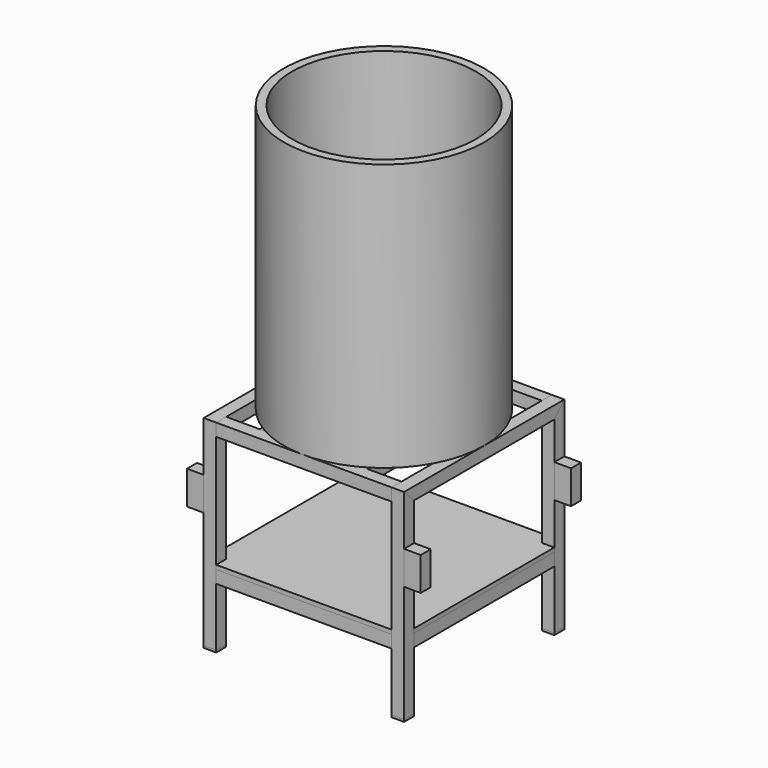
from build123d import *

# Parameters (mm, degrees)
F0_R           = 304.8
F1_DEPTH       = 812.8
F2_W           = 38.1
F2_H           = 38.1
F2_W_2         = 30.48
F2_H_2         = 30.48
F3_DEPTH       = 304.8
F5_DEPTH       = 38.1
F8_W           = 38.1
F8_H           = 38.1
F8_W_2         = 30.48
F8_H_2         = 30.48
F9_REACH       = 1476.2825367264
F12_W          = 38.1
F12_H          = 38.1
F12_W_2        = 30.48
F12_H_2        = 30.48
F13_DEPTH      = 266.7
F13_DEPTH_BACK = 266.7
F17_W          = 38.1
F17_H          = 38.1
F17_W_2        = 30.48
F17_H_2        = 30.48
F18_DEPTH      = 266.7
F18_DEPTH_BACK = 266.7
F20_W          = 38.1
F20_H          = 38.1
F20_W_2        = 30.48
F20_H_2        = 30.48
F21_DEPTH      = 266.7
F21_DEPTH_BACK = 266.7
F24_DEPTH      = 12.7
F25_W          = 38.1
F25_H          = 38.1
F25_R          = 6.35
F26_DEPTH      = 6.35
F29_R          = 279.4
F30_DEPTH      = 759.46
F31_W          = 38.1
F31_H          = 101.6
F32_DEPTH      = 50.8


with BuildPart() as f1:
    # F0 (on Top) → F1 (new body)
    with BuildSketch(Plane.XY):
        Circle(F0_R)
    extrude(amount=F1_DEPTH)

    # F29 (on face) → F30 (cut)
    with BuildSketch(Plane.XY.offset(812.8)):
        Circle(F29_R)
    extrude(amount=-F30_DEPTH, mode=Mode.SUBTRACT)


with BuildPart() as f3:
    # F2 (on Front) → F3 (new body, symmetric)
    with BuildSketch(Plane.XZ):
        with Locations((285.75, -19.05)):
            Rectangle(F2_W, F2_H)
        with Locations((285.75, -19.05)):
            Rectangle(F2_W_2, F2_H_2, mode=Mode.SUBTRACT)
    extrude(amount=F3_DEPTH, both=True)

    # F4 (on face) → F5 (cut, through all)
    with BuildSketch(Plane.YZ.offset(304.8)):
        Polygon((-266.7, -38.1), (-304.8, 0), (-315.9340023994, 0), (-315.9340023994, -51.912445575), (-266.7, -51.912445575), align=None)
        Polygon((315.9340023994, -51.912445575), (315.9340023994, 0), (304.8, 0), (266.7, -38.1), (266.7, -51.912445575), align=None)
    extrude(amount=-F5_DEPTH, mode=Mode.SUBTRACT)


with BuildPart() as f6_1:
    # F6: instance of F3
    add(f3.part.mirror(Plane.YZ))


with BuildPart() as f9:
    f9_end = f3.part.faces().sort_by_distance((285.75, -267.166627796, -37.633372204))[0]
    # F8 (on offset) → F9 (new body, up to a face of F3 that its end follows)
    with BuildSketch(Plane.XY.offset(-609.6)):
        with Locations((285.75, -285.75)):
            Rectangle(F8_W, F8_H)
        with Locations((285.75, -285.75)):
            Rectangle(F8_W_2, F8_H_2, mode=Mode.SUBTRACT)
    f9_long = extrude(amount=F9_REACH, mode=Mode.PRIVATE)
    add(split(f9_long, bisect_by=f9_end, keep=Keep.TOP, mode=Mode.PRIVATE))


with BuildPart() as f10_1:
    # F10: instance of F9
    add(f9.part.mirror(Plane.XZ))


with BuildPart() as f11_1:
    # F11: instance of F9
    add(f9.part.mirror(Plane.YZ))


with BuildPart() as f11_2:
    # F11: instance of F10_1
    add(f10_1.part.mirror(Plane.YZ))


with BuildPart() as f13:
    # F12 (on Right) → F13 (new body, two sides)
    with BuildSketch(Plane.YZ) as f13_sk:
        with Locations((-285.75, -19.05)):
            Rectangle(F12_W, F12_H)
        with Locations((-285.75, -19.05)):
            Rectangle(F12_W_2, F12_H_2, mode=Mode.SUBTRACT)
    extrude(amount=F13_DEPTH)
    extrude(f13_sk.sketch, amount=-F13_DEPTH_BACK)


with BuildPart() as f14_1:
    # F14: instance of F13
    add(f13.part.mirror(Plane.XZ))


with BuildPart() as f16_1:
    # F16: instance of F13
    add(f13.part.mirror(Plane(origin=(0, -285.75, -215.9), x_dir=(1, 0, 0), z_dir=(0, 0, -1))))


with BuildPart() as f16_2:
    # F16: instance of F14_1
    add(f14_1.part.mirror(Plane(origin=(0, -285.75, -215.9), x_dir=(1, 0, 0), z_dir=(0, 0, -1))))


with BuildPart() as f18:
    # F17 (on Front) → F18 (new body, two sides)
    with BuildSketch(Plane.XZ) as f18_sk:
        with Locations((285.75, -412.75)):
            Rectangle(F17_W, F17_H)
        with Locations((285.75, -412.75)):
            Rectangle(F17_W_2, F17_H_2, mode=Mode.SUBTRACT)
    extrude(amount=F18_DEPTH)
    extrude(f18_sk.sketch, amount=-F18_DEPTH_BACK)


with BuildPart() as f19_1:
    # F19: instance of F18
    add(f18.part.mirror(Plane.YZ))


with BuildPart() as f21:
    # F20 (on Front) → F21 (new body, two sides)
    with BuildSketch(Plane.XZ) as f21_sk:
        with Locations((-146.05, -19.05)):
            Rectangle(F20_W, F20_H)
        with Locations((-146.05, -19.05)):
            Rectangle(F20_W_2, F20_H_2, mode=Mode.SUBTRACT)
    extrude(amount=F21_DEPTH)
    extrude(f21_sk.sketch, amount=-F21_DEPTH_BACK)


with BuildPart() as f22_1:
    # F22: instance of F21
    add(f21.part.mirror(Plane.YZ))


with BuildPart() as f24:
    # F23 (on face) → F24 (new body)
    with BuildSketch(Plane.XY.offset(-393.7)):
        Polygon((-266.6999999998, -304.8), (266.7000000002, -304.8), (266.7, -266.7000000001), (304.8, -266.7000000001), (304.8, 266.7), (266.7, 266.7), (266.7000000002, 304.8), (-266.6999999998, 304.8), (-266.6999999998, 266.7), (-304.8, 266.7), (-304.8, -266.7000000001), (-266.7, -266.7000000001), align=None)
    extrude(amount=F24_DEPTH)


with BuildPart() as f26:
    # F25 (on offset) → F26 (new body)
    with BuildSketch(Plane.XY.offset(-609.6)):
        with Locations((285.75, -285.75)):
            Rectangle(F25_W, F25_H)
        with Locations((285.75, -285.75)):
            Circle(F25_R, mode=Mode.SUBTRACT)
    extrude(amount=-F26_DEPTH)


with BuildPart() as f27_1:
    # F27: instance of F26
    add(f26.part.mirror(Plane.YZ))


with BuildPart() as f28_1:
    # F28: instance of F26
    add(f26.part.mirror(Plane.XZ))


with BuildPart() as f28_2:
    # F28: instance of F27_1
    add(f27_1.part.mirror(Plane.XZ))


with BuildPart() as f32:
    # F31 (on face) → F32 (new body)
    with BuildSketch(Plane(origin=(-304.8, 0, 0), x_dir=(0, -1, 0), z_dir=(-1, 0, 0))):
        with Locations((-285.75, -203.2)):
            Rectangle(F31_W, F31_H)
    extrude(amount=F32_DEPTH)


with BuildPart() as f32b:
    # F31 (on face) → F32, piece 2 (new body)
    with BuildSketch(Plane(origin=(-304.8, 0, 0), x_dir=(0, -1, 0), z_dir=(-1, 0, 0))):
        with Locations((285.75, -203.2)):
            Rectangle(F31_W, F31_H)
    extrude(amount=F32_DEPTH)


with BuildPart() as f33_1:
    # F33: instance of F32b
    add(f32b.part.mirror(Plane.YZ))


with BuildPart() as f33_2:
    # F33: instance of F32
    add(f32.part.mirror(Plane.YZ))


solid = Compound([f1.part, f3.part, f6_1.part, f9.part, f10_1.part, f11_1.part, f11_2.part, f13.part, f14_1.part, f16_1.part, f16_2.part, f18.part, f19_1.part, f21.part, f22_1.part, f24.part, f26.part, f27_1.part, f28_1.part, f28_2.part, f32.part, f32b.part, f33_1.part, f33_2.part])
